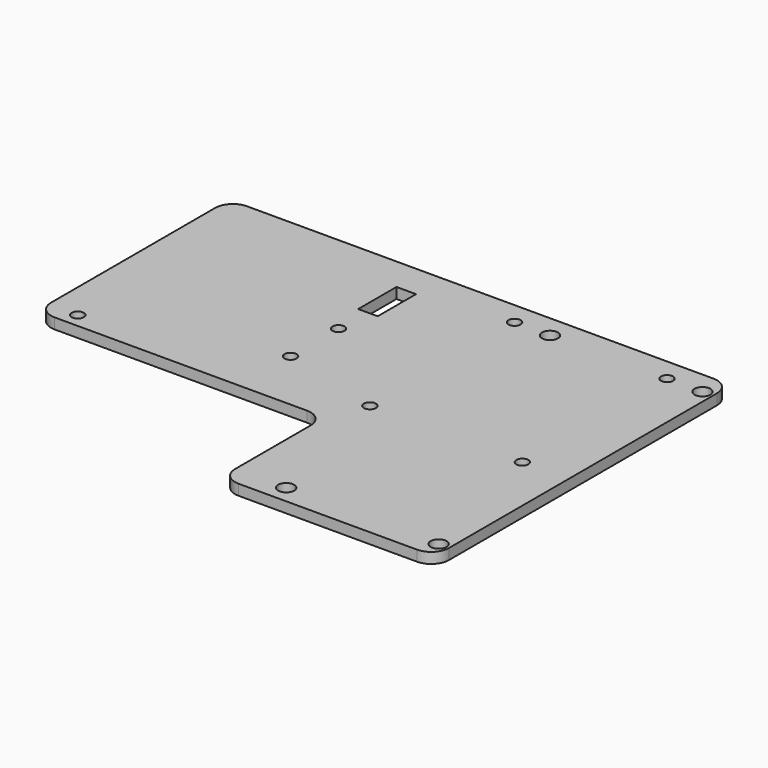
from build123d import *

# Parameters (mm, degrees)
F1_DEPTH = 3
F2_D     = 4.5
F3_R     = 5
F4_D     = 3.4
F6_D     = 3.4
F5_W     = 5.5
F5_H     = 13.5
F7_DEPTH = 25


# Not quite as in the source:
# - a feature names something its author has since deleted; it is built from what else it names


with BuildPart() as f1:
    # F0 (on Top) → F1 (new body)
    with BuildSketch(Plane.XY):
        Polygon((-35.8541943133, -51.5685416758), (24.4538411498, -51.5685416758), (24.4538411498, 52.9103763402), (-117.0655786991, 52.9103763402), (-117.0655786991, -14.937300235), (-35.8541943133, -14.937300235), align=None)
    extrude(amount=F1_DEPTH)

    # F2 (through all)
    with Locations(Plane(origin=(0, 0, 0), x_dir=(1, 0, 0), z_dir=(0, 0, -1))):
        with Locations((-21.5, -46.5), (21.5, -46.5), (21.5, 46.5), (-21.5, 46.5)):
            Hole(F2_D / 2)

    # F3
    f3_edges = [f1.edges().sort_by_distance(p)[0] for p in [
        (-117.065579, 52.910376, 1.5),
        (24.453841, 52.910376, 1.5),
        (24.453841, -51.568542, 1.5),
        (-35.854194, -14.9373, 1.5),
        (-35.854194, -51.568542, 1.5),
        (-117.065579, -14.9373, 1.5),
    ]]
    fillet(f3_edges, radius=F3_R)

    # F4 (through all)
    with Locations(Plane(origin=(0, 0, 0), x_dir=(1, 0, 0), z_dir=(0, 0, -1))):
        with Locations((-31.5, -46.5), (11.5, -46.5), (11.5, 4.5), (-31.5, 4.5)):
            Hole(F4_D / 2)

    # F6 (through all)
    with Locations(Plane.XY.offset(3)):
        with Locations((-59.8872532725, 3.0199595654), (-59.8872532725, 19.9299595654), (-108.7842532725, -10.8700404346)):
            Hole(F6_D / 2)

    # F5 (on face) → F7 (cut)
    with BuildSketch(Plane.XY.offset(3)):
        with Locations((-59.5872532725, 36.6799595654)):
            Rectangle(F5_W, F5_H)
    extrude(amount=-F7_DEPTH, mode=Mode.SUBTRACT)


solid = f1.part
